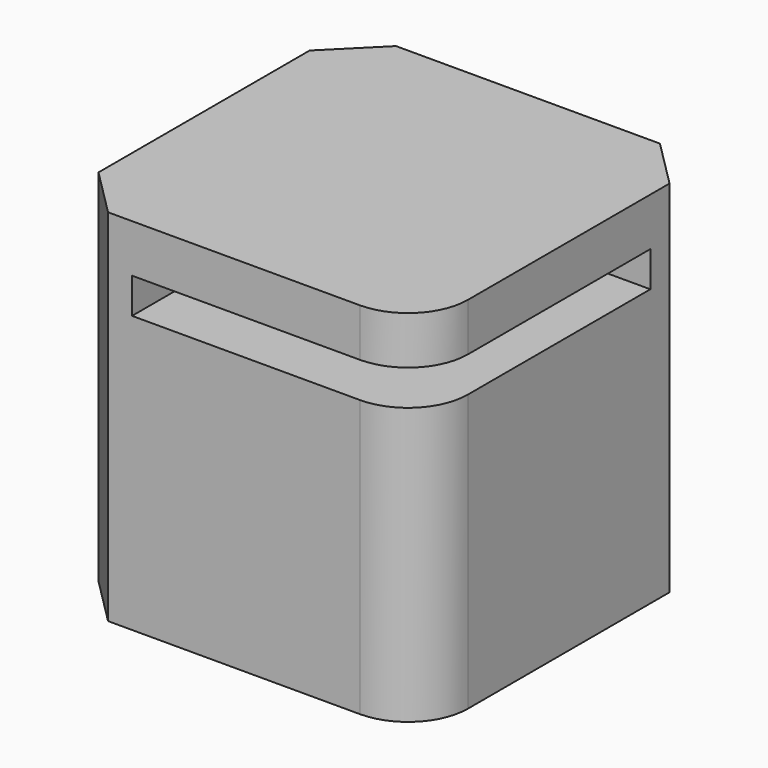
from build123d import *

# Parameters (mm, degrees)
F0_W     = 15
F0_H     = 15
F1_DEPTH = 15
F2_W     = 12
F2_H     = 1.475
F3_DEPTH = 12
F4_R     = 5
F5_R     = 7
F6_DEPTH = 3.2
F7_SIZE2 = 3.19999
F7_SIZE  = 2.49999
F8_R     = 2.5
F9_SIZE  = 2


# Not quite as in the source:
# - a fillet or chamfer is up to 0.001 mm smaller than in the source, because OpenCascade refuses the exact size


with BuildPart() as f1:
    # F0 (on Top) → F1 (new body)
    with BuildSketch(Plane.XY):
        with Locations((7.5, 7.5)):
            Rectangle(F0_W, F0_H)
    extrude(amount=F1_DEPTH)

    # F2 (on face) → F3 (cut)
    with BuildSketch(Plane.XZ):
        with Locations((9, 12.2625)):
            Rectangle(F2_W, F2_H)
    extrude(amount=-F3_DEPTH, mode=Mode.SUBTRACT)

    # F4
    f4_edges = [f1.edges().sort_by_distance(p)[0] for p in [
        (3, 12, 12.2625),
    ]]
    fillet(f4_edges, radius=F4_R)

    # F5 (on face) → F6 (cut)
    with BuildSketch(Plane(origin=(0, 0, 0), x_dir=(1, 0, 0), z_dir=(0, 0, -1))):
        with Locations((7.5, -7.5)):
            Circle(F5_R)
    extrude(amount=-F6_DEPTH, mode=Mode.SUBTRACT)

    # F7 (size 2.5 and 3.2 in the source; OpenCascade refuses exactly that, so slightly less here)
    f7_edges = [f1.edges().sort_by_distance(p)[0] for p in [
        (0.5, 7.5, 3.2),
    ]]
    f7_side = f1.faces().sort_by_distance((7.5, 7.5, 3.2))[0]
    chamfer(f7_edges, length=F7_SIZE, length2=F7_SIZE2, reference=f7_side)

    # F8
    f8_edges = [f1.edges().sort_by_distance(p)[0] for p in [
        (15, 0, 14),
        (15, 0, 5.7625),
    ]]
    fillet(f8_edges, radius=F8_R)

    # F9
    f9_edges = [f1.edges().sort_by_distance(p)[0] for p in [
        (15, 15, 7.5),
        (0, 15, 7.5),
        (0, 0, 7.5),
    ]]
    chamfer(f9_edges, length=F9_SIZE)


solid = f1.part
